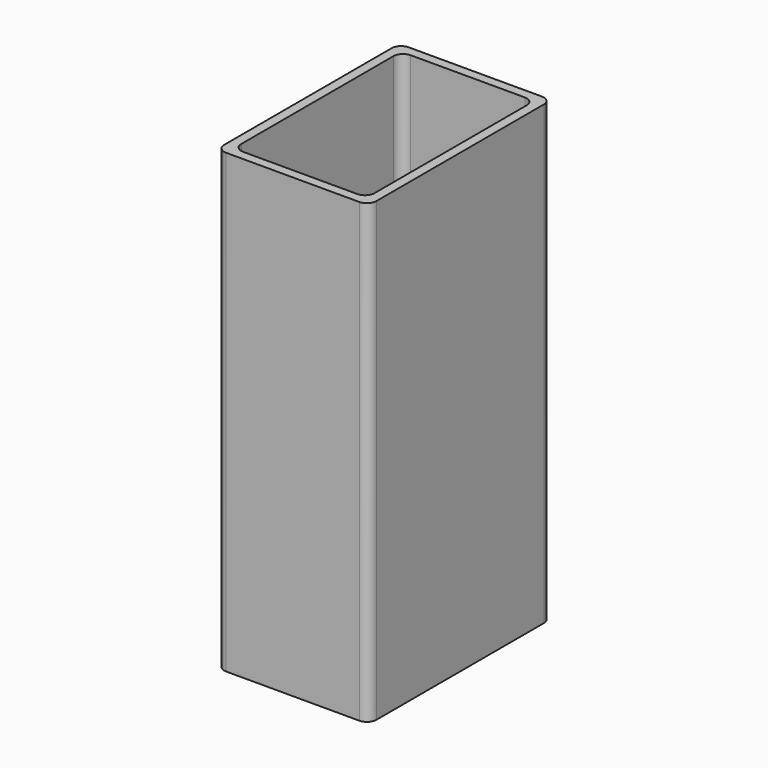
from build123d import *

# Parameters (mm, degrees)
F0_W     = 50.8
F0_H     = 76.2
F0_W_2   = 44.45
F0_H_2   = 69.85
F2_DEPTH = 152.4
F3_R     = 3.175


# Not quite as in the source:
# - a variable given as a bare number and used for a length is read in inches; the dataset says mm whatever the document's units were


with BuildPart() as f2:
    # F0 (on Top) → F2 (new body)
    with BuildSketch(Plane.XY):
        Rectangle(F0_W, F0_H)
        Rectangle(F0_W_2, F0_H_2, mode=Mode.SUBTRACT)
    extrude(amount=F2_DEPTH)

    # F3
    f3_edges = [f2.edges().sort_by_distance(p)[0] for p in [
        (-22.225, 34.925, 76.2),
        (22.225, 34.925, 76.2),
        (22.225, -34.925, 76.2),
        (-22.225, -34.925, 76.2),
        (25.4, 38.1, 76.2),
        (-25.4, 38.1, 76.2),
        (25.4, -38.1, 76.2),
        (-25.4, -38.1, 76.2),
    ]]
    fillet(f3_edges, radius=F3_R)


solid = f2.part
